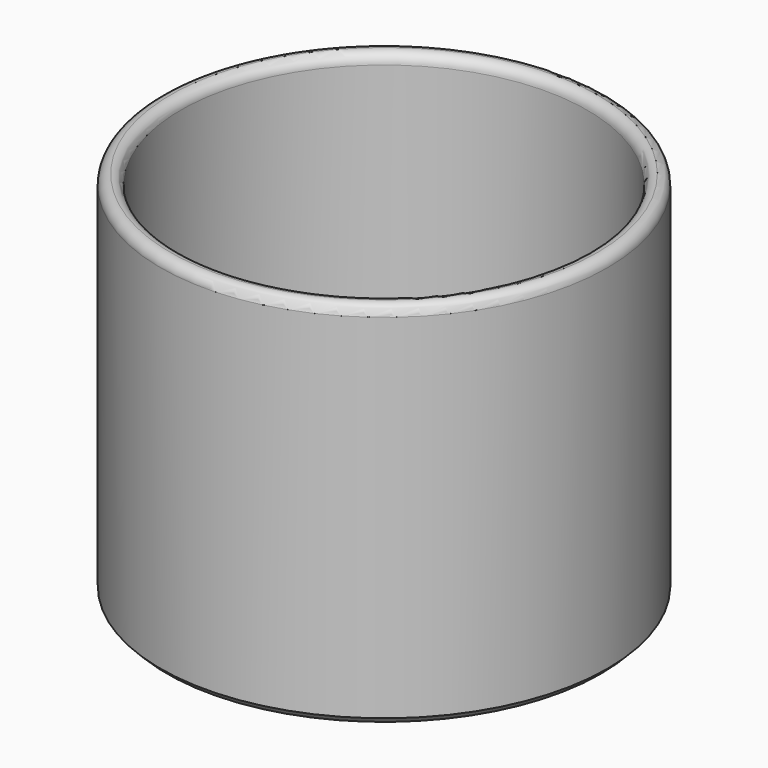
from build123d import *

# Parameters (mm, degrees)
F2_R    = 2.99999
F3_R    = 2.99999
F4_R    = 1.49999
F5_SIZE = 1


# Not quite as in the source:
# - a fillet or chamfer is up to 0.001 mm smaller than in the source, because OpenCascade refuses the exact size


with BuildPart() as f1:
    # F0 (on Front) → F1 (revolve)
    with BuildSketch(Plane.XZ):
        Polygon((30.25, 0), (33.25, 0), (33.25, 55), (30.25, 55), (30.25, 17), (27.25, 17), (27.25, 15), (30.25, 15), align=None)
    revolve(axis=Axis((0, 0, 28.8916025311), (0, 0, 1)))

    # F2 (radius 3 in the source; OpenCascade refuses exactly that, so slightly less here)
    f2_edges = [f1.edges().sort_by_distance(p)[0] for p in [
        (-30.25, 0, 17),
    ]]
    fillet(f2_edges, radius=F2_R)

    # F3 (radius 3 in the source; OpenCascade refuses exactly that, so slightly less here)
    f3_edges = [f1.edges().sort_by_distance(p)[0] for p in [
        (-30.25, 0, 15),
    ]]
    fillet(f3_edges, radius=F3_R)

    # F4 (radius 1.5 in the source; OpenCascade refuses exactly that, so slightly less here)
    f4_edges = [f1.edges().sort_by_distance(p)[0] for p in [
        (-30.25, 0, 55),
        (-33.25, 0, 55),
    ]]
    fillet(f4_edges, radius=F4_R)

    # F5
    f5_edges = [f1.edges().sort_by_distance(p)[0] for p in [
        (-33.25, 0, 0),
    ]]
    chamfer(f5_edges, length=F5_SIZE)


solid = f1.part
